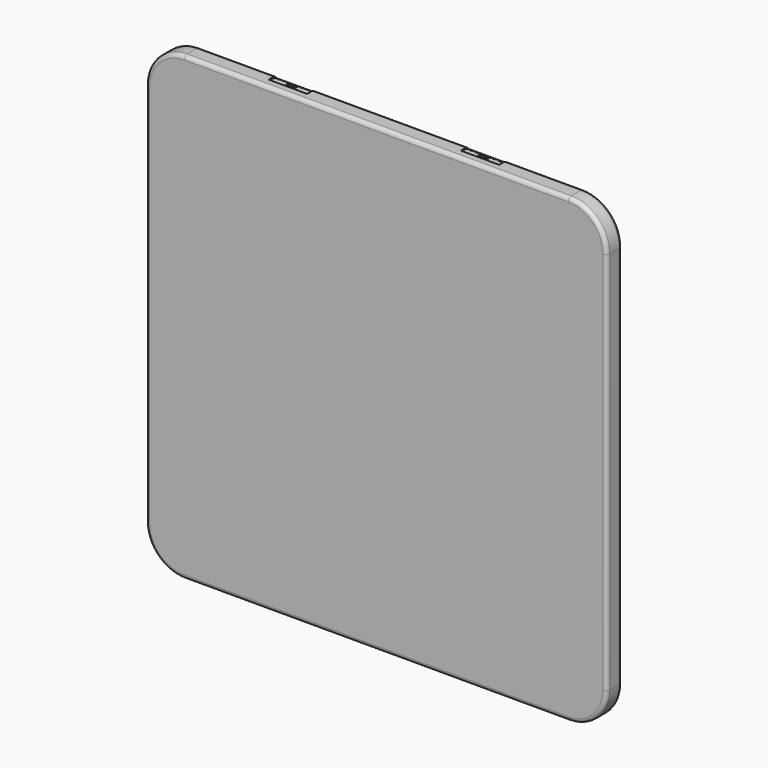
from build123d import *

# Parameters (mm, degrees)
F0_W         = 609.6
F0_H         = 609.6
F1_DEPTH     = 25.4
F2_R         = 50.8
F4_DEPTH     = 12.7
F6_DEPTH     = 50.8
F7_DEPTH     = 19.05
F9_DEPTH     = 19.05
F10_W        = 50.8
F10_H        = 1.27
F11_DEPTH    = 12.7
F13_DEPTH    = 1.27
F14_T1_DEPTH = 50.292
F15_R        = 5.08
F17_DEPTH    = 50.8
F18_DEPTH    = 19.05
F19_R        = 5.08
F19_R_2      = 3.81
F20_DEPTH    = 19.05
F21_W        = 50.8
F21_H        = 12.7
F22_DEPTH    = 1.27
F23_W        = 50.292
F23_H        = 22.86
F24_DEPTH    = 1.27
F25_T1_DEPTH = 50.292
F27_DEPTH    = 50.8
F29_DEPTH    = 50.8
F31_DEPTH    = 12.7
F33_DEPTH    = 12.7
F34_W        = 12.7
F34_H        = 39.37
F35_DEPTH    = 2.54
F37_DEPTH    = 10.414
F38_R        = 3.175
F39_DEPTH    = 50.8
F40_R        = 3.81
F41_DEPTH    = 12.7
F38_R_2      = 3.81
F42_DEPTH    = 12.7
F43_DEPTH    = 1.27


# Not quite as in the source:
# - a fillet or chamfer that OpenCascade refuses, or shapes differently, is made with other operations: its cross-section is extruded or revolved along the edge and cut away or added


with BuildPart() as f1:
    # F0 (on Front) → F1 (new body)
    with BuildSketch(Plane.XZ):
        Rectangle(F0_W, F0_H)
    extrude(amount=F1_DEPTH)

    # F2
    f2_edges = [f1.edges().sort_by_distance(p)[0] for p in [
        (304.8, -12.7, 304.8),
        (-304.8, -12.7, 304.8),
        (-304.8, -12.7, -304.8),
        (304.8, -12.7, -304.8),
    ]]
    fillet(f2_edges, radius=F2_R)

    # F3 (on face) → F4 (cut)
    with BuildSketch(Plane.XY.offset(304.8)):
        Polygon((-101.6, -12.7), (-101.6, 0), (-127, 0), (-152.4, 0), (-152.4, -12.7), align=None)
        Polygon((127, 0), (101.6, 0), (101.6, -12.7), (152.4, -12.7), (152.4, 0), align=None)
    extrude(amount=-F4_DEPTH, mode=Mode.SUBTRACT)

    # F5 (on face) → F6 (join)
    with BuildSketch(Plane.YZ.offset(-152.4)):
        with BuildLine():
            ThreePointArc((-3.2004, 298.45), (-6.3754, 301.625), (-9.5504, 298.45))
            ThreePointArc((-9.5504, 298.45), (-6.3754, 295.275), (-3.2004, 298.45))
        make_face()
    extrude(amount=F6_DEPTH)

    # F5 (on face) → F7 (join)
    with BuildSketch(Plane.YZ.offset(-152.4)):
        with BuildLine():
            ThreePointArc((-1.2954, 298.45), (-6.3754, 303.53), (-11.4554, 298.45))
            ThreePointArc((-11.4554, 298.45), (-6.3754, 293.37), (-1.2954, 298.45))
        make_face()
        with BuildLine():
            ThreePointArc((-2.5654, 298.45), (-6.3754, 294.64), (-10.1854, 298.45))
            ThreePointArc((-10.1854, 298.45), (-6.3754, 302.26), (-2.5654, 298.45))
        make_face(mode=Mode.SUBTRACT)
    extrude(amount=F7_DEPTH)

    # F8 (on face) → F9 (join)
    with BuildSketch(Plane(origin=(-101.6, 0, 0), x_dir=(0, -1, 0), z_dir=(-1, 0, 0))):
        with BuildLine():
            ThreePointArc((11.4554, 298.45), (6.3754, 303.53), (1.2954, 298.45))
            ThreePointArc((1.2954, 298.45), (6.3754, 293.37), (11.4554, 298.45))
        make_face()
        with BuildLine():
            ThreePointArc((10.1854, 298.45), (6.3754, 294.64), (2.5654, 298.45))
            ThreePointArc((2.5654, 298.45), (6.3754, 302.26), (10.1854, 298.45))
        make_face(mode=Mode.SUBTRACT)
    extrude(amount=F9_DEPTH)

    # F10 (on face) → F11 (cut)
    with BuildSketch(Plane.XY.offset(292.1)):
        with Locations((-127, -0.635)):
            Rectangle(F10_W, F10_H)
    extrude(amount=-F11_DEPTH, mode=Mode.SUBTRACT)

    # F12 (on face) → F13 (join)
    with BuildSketch(Plane(origin=(0, -1.27, 0), x_dir=(-1, 0, 0), z_dir=(0, 1, 0))):
        Polygon((101.854, 302.26), (101.854, 279.654), (127.4700760841, 279.654), (152.146, 279.654), (152.146, 302.26), align=None)
    extrude(amount=F13_DEPTH)

    # F14: fillet of radius 2.54 on 1 edges, made by hand

    # F14_s2 → F14_t1 (cut)
    with BuildSketch(Plane.YZ.offset(-152.146)):
        with BuildLine():
            ThreePointArc((-1.269799924, 302.2603463663), (-0.3399390393, 301.3301793667), (0.0004, 300.0597380063))
            Line((0.0004, 300.0597380063), (0.2545365685, 300.0597380063))
            ThreePointArc((0.2545365685, 300.0597380063), (0.2541365685, 301.1598690031), (0.2541365685, 302.26))
            Line((0.2541365685, 302.26), (0, 302.5141365685))
            ThreePointArc((0, 302.5141365685), (-0.634899962, 302.5141365685), (-1.1426833478, 302.4804072023))
            Line((-1.1426833478, 302.4804072023), (-1.269799924, 302.2603463663))
        make_face()
    extrude(amount=F14_T1_DEPTH, mode=Mode.SUBTRACT)

    # F15
    f15_edges = [f1.edges().sort_by_distance(p)[0] for p in [
        (-304.8, 0, 0),
        (-304.8, -25.4, 0),
        (-289.921024, -25.4, 289.921024),
        (-289.921024, 0, 289.921024),
        (0, 0, 304.8),
        (304.8, 0, 0),
        (304.8, -25.4, 0),
        (289.921024, 0, -289.921024),
        (289.921024, 0, 289.921024),
        (203.2, 0, 304.8),
        (-203.2, 0, 304.8),
        (-289.921024, 0, -289.921024),
        (0, 0, -304.8),
        (289.921024, -25.4, -289.921024),
        (289.921024, -25.4, 289.921024),
        (0, -25.4, -304.8),
        (0, -25.4, 304.8),
        (-289.921024, -25.4, -289.921024),
    ]]
    fillet(f15_edges, radius=F15_R)

    # F16 (on face) → F17 (join)
    with BuildSketch(Plane.YZ.offset(101.6)):
        with BuildLine():
            ThreePointArc((-3.2004, 298.45), (-6.3754, 301.625), (-9.5504, 298.45))
            ThreePointArc((-9.5504, 298.45), (-6.3754, 295.275), (-3.2004, 298.45))
        make_face()
    extrude(amount=F17_DEPTH)

    # F16 (on face) → F18 (join)
    with BuildSketch(Plane.YZ.offset(101.6)):
        with BuildLine():
            ThreePointArc((-1.2954, 298.45), (-6.3754, 303.53), (-11.4554, 298.45))
            ThreePointArc((-11.4554, 298.45), (-6.3754, 293.37), (-1.2954, 298.45))
        make_face()
        with BuildLine():
            ThreePointArc((-2.5654, 298.45), (-6.3754, 294.64), (-10.1854, 298.45))
            ThreePointArc((-10.1854, 298.45), (-6.3754, 302.26), (-2.5654, 298.45))
        make_face(mode=Mode.SUBTRACT)
    extrude(amount=F18_DEPTH)

    # F19 (on face) → F20 (join)
    with BuildSketch(Plane(origin=(152.4, 0, 0), x_dir=(0, -1, 0), z_dir=(-1, 0, 0))):
        with Locations((6.3754, 298.45)):
            Circle(F19_R)
        with Locations((6.3754, 298.45)):
            Circle(F19_R_2, mode=Mode.SUBTRACT)
    extrude(amount=F20_DEPTH)

    # F21 (on face) → F22 (cut)
    with BuildSketch(Plane(origin=(0, 0, 0), x_dir=(-1, 0, 0), z_dir=(0, 1, 0))):
        with Locations((-127, 285.75)):
            Rectangle(F21_W, F21_H)
    extrude(amount=-F22_DEPTH, mode=Mode.SUBTRACT)

    # F23 (on face) → F24 (join)
    with BuildSketch(Plane(origin=(0, -1.27, 0), x_dir=(-1, 0, 0), z_dir=(0, 1, 0))):
        with Locations((-127, 291.084)):
            Rectangle(F23_W, F23_H)
    extrude(amount=F24_DEPTH)

    # F25: fillet of radius 2.54 on 1 edges, made by hand

    # F25_s2 → F25_t1 (cut)
    with BuildSketch(Plane.YZ.offset(101.854)):
        with BuildLine():
            ThreePointArc((-1.27, 302.514), (-0.3402954744, 301.5842954744), (0, 300.3142954744))
            Line((0, 300.3142954744), (0, 302.514))
            Line((0, 302.514), (-1.27, 302.514))
        make_face()
    extrude(amount=F25_T1_DEPTH, mode=Mode.SUBTRACT)

    # F26 (on face) → F27 (join)
    with BuildSketch(Plane.YZ.offset(101.6)):
        with BuildLine():
            Line((-1.27, 299.339), (-1.27, 302.514))
            Line((-1.27, 302.514), (-3.302, 302.514))
            ThreePointArc((-3.302, 302.514), (-1.9806035483, 301.1219537291), (-1.27, 299.339))
        make_face()
    extrude(amount=F27_DEPTH)

    # F28 (on face) → F29 (join)
    with BuildSketch(Plane.YZ.offset(-152.4)):
        with BuildLine():
            Line((-1.27, 299.085), (-1.27, 302.26))
            Line((-1.27, 302.26), (-3.048, 302.26))
            ThreePointArc((-3.048, 302.26), (-1.8649538604, 300.8371658382), (-1.27, 299.085))
        make_face()
    extrude(amount=F29_DEPTH)

    # F30 (on face) → F31 (cut)
    with BuildSketch(Plane(origin=(0, 0, 0), x_dir=(-1, 0, 0), z_dir=(0, 1, 0))):
        Polygon((-253.6922354202, 289.6132599045), (-271.6527476623, 271.6527476623), (-289.6132599045, 253.6922354202), (253.6922354202, -289.6132599045), (271.6527476623, -271.6527476623), (289.6132599045, -253.6922354202), align=None)
    extrude(amount=-F31_DEPTH, mode=Mode.SUBTRACT)

    # F32 (on face) → F33 (join)
    with BuildSketch(Plane(origin=(0, -12.7, 0), x_dir=(-1, 0, 0), z_dir=(0, 1, 0))):
        Polygon((-250.3770757206, 281.8079721443), (-253.6922354202, 285.1231318439), (-258.918592355, 279.8967749092), (-285.1231318439, 253.6922354202), (-222.135802757, 190.7049063332), (253.6922354202, -285.1231318439), (270.6703651647, -268.1450020994), (285.1231318439, -253.6922354202), align=None)
    extrude(amount=F33_DEPTH)

    # F34 (on face) → F35 (join)
    with BuildSketch(Plane(origin=(269.4076836321, 0, 269.4076836321), x_dir=(0, 1, 0), z_dir=(0.7071067812, 0, 0.7071067812))):
        with Locations((-6.35, 0)):
            Rectangle(F34_W, F34_H)
    extrude(amount=F35_DEPTH)

    # F36 (on face) → F37 (cut)
    with BuildSketch(Plane(origin=(0, 0, 0), x_dir=(-1, 0, 0), z_dir=(0, 1, 0))):
        Polygon((-292.4869418632, 264.6481478879), (-285.9313548948, 258.0925609195), (-258.0925609195, 285.9313548948), (-264.6481478879, 292.4869418632), align=None)
        Polygon((-258.0925609195, 285.9313548948), (-285.9313548948, 258.0925609195), (-285.57214465, 257.7333506747), (-257.7333506747, 285.57214465), align=None)
    extrude(amount=-F37_DEPTH, mode=Mode.SUBTRACT)

    # F38 (on face) → F39 (join)
    with BuildSketch(Plane(origin=(-13.9193969877, 0, 13.9193969877), x_dir=(0.7071067812, 0, 0.7071067812), z_dir=(0.7071067812, 0, -0.7071067812))):
        with Locations((388.62, 5.207)):
            Circle(F38_R)
    extrude(amount=F39_DEPTH)

    # F40 (on face) → F41 (join)
    with BuildSketch(Plane(origin=(13.9193969877, 0, -13.9193969877), x_dir=(0.7071067812, 0, 0.7071067812), z_dir=(-0.7071067812, 0, 0.7071067812))):
        with BuildLine():
            ThreePointArc((384.175, -7.6663444248), (389.89, -10.1256888497), (393.7, -5.207))
            ThreePointArc((393.7, -5.207), (389.89, -0.2883111503), (384.175, -2.7476555752))
            Line((384.175, -2.7476555752), (384.175, -7.6663444248))
        make_face()
        with Locations((388.62, -5.207)):
            Circle(F40_R, mode=Mode.SUBTRACT)
    extrude(amount=F41_DEPTH)

    # F38 (on face) → F42 (join)
    with BuildSketch(Plane(origin=(-13.9193969877, 0, 13.9193969877), x_dir=(0.7071067812, 0, 0.7071067812), z_dir=(0.7071067812, 0, -0.7071067812))):
        with BuildLine():
            ThreePointArc((384.175, 2.7476555752), (389.89, 0.2883111503), (393.7, 5.207))
            ThreePointArc((393.7, 5.207), (389.89, 10.1256888497), (384.175, 7.6663444248))
            Line((384.175, 7.6663444248), (384.175, 2.7476555752))
        make_face()
        with Locations((388.62, 5.207)):
            Circle(F38_R_2, mode=Mode.SUBTRACT)
    extrude(amount=F42_DEPTH)

    # F43 (add): a face of the model
    f43_faces = [f1.faces().sort_by_distance(p)[0] for p in [
        (271.2037348563, -6.35, 271.2037348563),
    ]]
    extrude(f43_faces, amount=F43_DEPTH)


solid = f1.part
